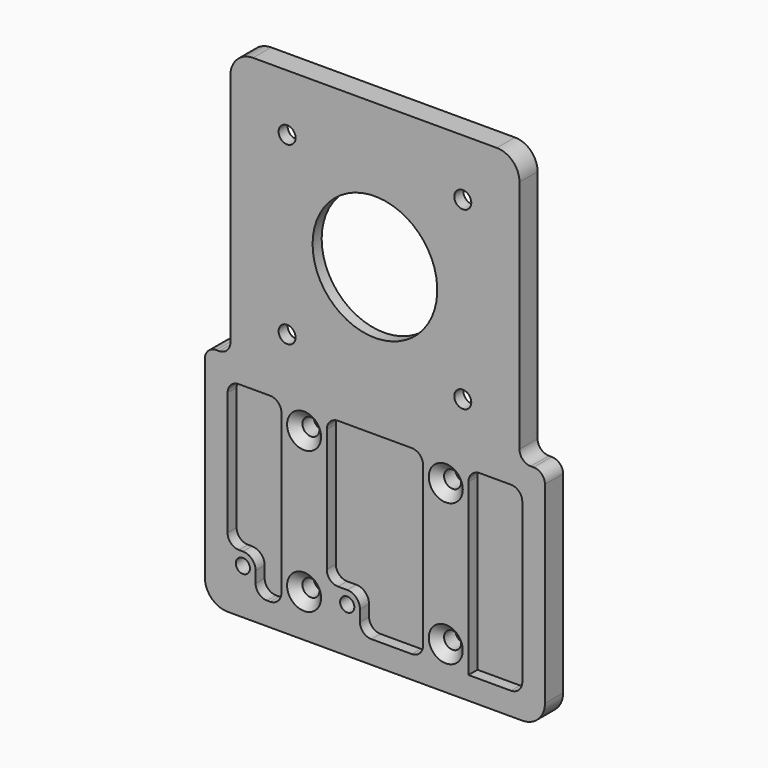
from build123d import *

# Parameters (mm, degrees)
F0_W           = 51
F0_H           = 47.5
F1_DEPTH       = 4
F2_W           = 43
F2_H           = 43
F2_R           = 11
F3_DEPTH       = 2
F4_DEPTH       = 4.001
F5_D           = 3
F6_R           = 2
F7_W           = 9.5
F7_H           = 32
F8_DEPTH       = 2
F9_D           = 3
F9_CSINK_D     = 6
F9_CSINK_ANGLE = 90
F10_D          = 2.5
F11_R          = 2
F13_R          = 4


# Not quite as in the source:
# - two fillets or chamfers of one size are made in one step
# - a pattern or mirror of a feature is missing from the dataset's text; its kind, count and spacing are read off the source's solid


with BuildPart() as f1:
    # F0 (on Front) → F1 (new body)
    with BuildSketch(Plane.XZ):
        Polygon((25.5, -2), (-25.5, -2), (-30, -2), (-30, -42), (30, -42), (30, -2), align=None)
        with Locations((0, 21.75)):
            Rectangle(F0_W, F0_H)
    extrude(amount=F1_DEPTH)

    # F2 (on face) → F3 (cut)
    with BuildSketch(Plane(origin=(0, 0, 0), x_dir=(-1, 0, 0), z_dir=(0, 1, 0))):
        with Locations((0, 20)):
            Rectangle(F2_W, F2_H)
        with Locations((0, 20)):
            Circle(F2_R, mode=Mode.SUBTRACT)
    extrude(amount=-F3_DEPTH, mode=Mode.SUBTRACT)

    # F2 (on face) → F4 (cut, through all)
    with BuildSketch(Plane(origin=(0, 0, 0), x_dir=(-1, 0, 0), z_dir=(0, 1, 0))):
        with Locations((0, 20)):
            Circle(F2_R)
    extrude(amount=-F4_DEPTH, mode=Mode.SUBTRACT)

    # F5 (through all)
    with Locations(Plane(origin=(0, 0, 0), x_dir=(-1, 0, 0), z_dir=(0, 1, 0))):
        with Locations((-15.5, 35.5), (15.5, 35.5), (15.5, 4.5), (-15.5, 4.5)):
            Hole(F5_D / 2)

    # F6
    f6_edges = [f1.edges().sort_by_distance(p)[0] for p in [
        (21.5, -1, 41.5),
        (-21.5, -1, 41.5),
        (-21.5, -1, -1.5),
        (21.5, -1, -1.5),
    ]]
    fillet(f6_edges, radius=F6_R)

    # F7 (on face) → F8 (cut)
    with BuildSketch(Plane.XZ.offset(4)):
        with BuildLine():
            Line((-16.5, -38), (-16.5, -6))
            Line((-16.5, -6), (-26, -6))
            Line((-26, -6), (-26, -31.75))
            Line((-26, -31.75), (-23.3, -31.75))
            ThreePointArc((-23.3, -31.75), (-21.7090097423, -32.4090097423), (-21.05, -34))
            Line((-21.05, -34), (-21.05, -38))
            Line((-21.05, -38), (-16.5, -38))
        make_face()
        with BuildLine():
            Line((8.5, -38), (8.5, -6))
            Line((8.5, -6), (-8.5, -6))
            Line((-8.5, -6), (-8.5, -31.75))
            Line((-8.5, -31.75), (-4.89, -31.75))
            ThreePointArc((-4.89, -31.75), (-3.2990097423, -32.4090097423), (-2.64, -34))
            Line((-2.64, -34), (-2.64, -38))
            Line((-2.64, -38), (8.5, -38))
        make_face()
        with Locations((21.25, -22)):
            Rectangle(F7_W, F7_H)
    extrude(amount=-F8_DEPTH, mode=Mode.SUBTRACT)

    # F9 (through all)
    with Locations(Plane.XZ.offset(4)):
        with Locations((-12.5, -9.5), (-12.5, -9.5), (-12.5, -34.5), (12.5, -34.5)):
            f9 = CounterSinkHole(F9_D / 2, F9_CSINK_D / 2, counter_sink_angle=F9_CSINK_ANGLE)

    # F9_copies: F9 across plane
    add(f9.mirror(Plane(origin=(0, 0, 0), x_dir=(0, 0, 1), z_dir=(1, 0, 0))), mode=Mode.SUBTRACT)

    # F10 (through all)
    with Locations(Plane.XZ.offset(4)):
        with Locations((-23.3, -34), (-4.89, -34)):
            Hole(F10_D / 2)

    # F11
    f11_edges = [f1.edges().sort_by_distance(p)[0] for p in [
        (-26, -3, -6),
        (26, -3, -6),
        (26, -3, -38),
        (-16.5, -3, -38),
        (8.5, -3, -38),
        (-16.5, -3, -6),
        (8.5, -3, -6),
        (-8.5, -3, -6),
        (16.5, -3, -6),
        (-8.5, -3, -31.75),
        (-25.5, -2, -2),
        (-30, -2, -2),
        (25.5, -2, -2),
        (30, -2, -2),
        (-21.05, -3, -38),
        (-26, -3, -31.75),
        (-2.64, -3, -38),
    ]]
    fillet(f11_edges, radius=F11_R)

    # F13
    f13_edges = [f1.edges().sort_by_distance(p)[0] for p in [
        (25.5, -2, 45.5),
        (-25.5, -2, 45.5),
        (-30, -2, -42),
        (30, -2, -42),
    ]]
    fillet(f13_edges, radius=F13_R)


solid = f1.part
